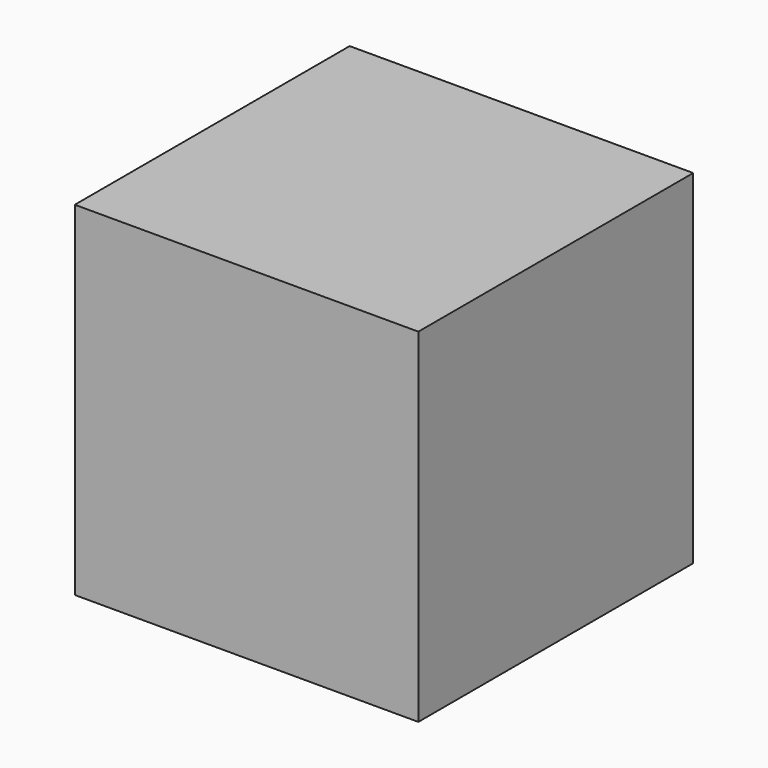
from build123d import *

# Parameters (mm, degrees)
F1_E0_W  = 1000
F1_E0_H  = 1000
F2_DEPTH = 1000


with BuildPart() as f2:
    # F1_E0 (on explicit) → F2 (new body)
    with BuildSketch(Plane.XY):
        with Locations((500, 500)):
            Rectangle(F1_E0_W, F1_E0_H)
    extrude(amount=F2_DEPTH)


solid = f2.part
